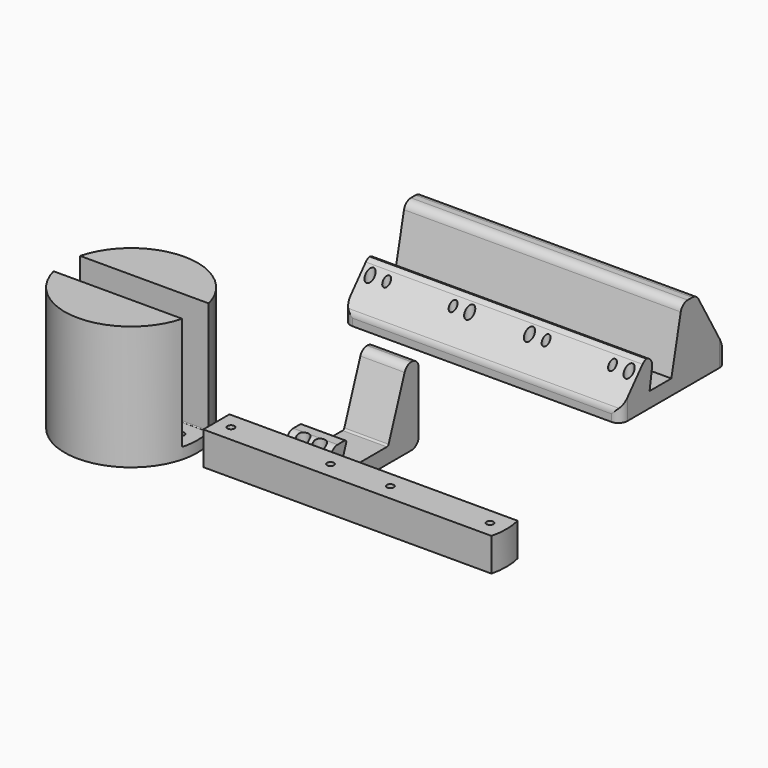
from build123d import *

# Parameters (mm, degrees)
F0_R            = 38.1
F1_DEPTH        = 71.12
F3_DEPTH        = 64.77
F4_R            = 2
F5_DEPTH        = 3.5
F5_FACE_R       = 2
F6_DEPTH        = 25.4
F7_R            = 2
F8_DEPTH        = 3.5
F9_DEPTH        = 6.351
F10_R           = 0.508
F11_R           = 2
F12_DEPTH       = 19.05
F13_W           = 158.75
F13_H           = 76.2
F13_R           = 2.5
F13_R_2         = 2
F14_DEPTH       = 6
F16_DEPTH       = 158.75
F17_T1_DEPTH    = 168.2889113945
F17_T3_DEPTH    = 170.280744219
F17_T5_DEPTH    = 31.4
F17_T7_DEPTH    = 165.5459461939
F17_T9_DEPTH    = 173.4270951792
F17_T11_DEPTH   = 179.186662319
F17_T13_DEPTH   = 188.398497554
F18_DEPTH       = 65.1210001
F20_DEPTH       = 25.4
F21_R           = 5.08
F22_R           = 1.27
F25_D           = 3.5
F25_DEPTH       = 25.4
F25_START       = 7.9337086
F25_CBORE_D     = 7
F25_CBORE_DEPTH = 7.112
F25_TIP         = 1.0515060833


# Not quite as in the source:
# - a fillet or chamfer that OpenCascade refuses, or shapes differently, is made with other operations: its cross-section is extruded or revolved along the edge and cut away or added


with BuildPart() as f1:
    # F0 (on Top) → F1 (new body)
    with BuildSketch(Plane.XY):
        with Locations((-43.8732802868, -98.4302014112)):
            Circle(F0_R)
    extrude(amount=F1_DEPTH)

    # F2 (on face) → F3 (cut)
    with BuildSketch(Plane.XY.offset(71.12)):
        with BuildLine():
            Line((-6.9831139142, -88.9052014112), (-80.7634466594, -88.9052014112))
            ThreePointArc((-80.7634466594, -88.9052014112), (-81.6696117146, -93.6294378677), (-81.9732802868, -98.4302014112))
            ThreePointArc((-81.9732802868, -98.4302014112), (-81.6696117146, -103.2309649548), (-80.7634466594, -107.9552014112))
            Line((-80.7634466594, -107.9552014112), (-6.9831139142, -107.9552014112))
            ThreePointArc((-6.9831139142, -107.9552014112), (-6.076948859, -103.2309649548), (-5.7732802868, -98.4302014112))
            ThreePointArc((-5.7732802868, -98.4302014112), (-6.076948859, -93.6294378677), (-6.9831139142, -88.9052014112))
        make_face()
    extrude(amount=-F3_DEPTH, mode=Mode.SUBTRACT)

    # F4 (on face) → F5 (cut)
    with BuildSketch(Plane(origin=(0, 0, 0), x_dir=(1, 0, 0), z_dir=(0, 0, -1))):
        Polygon((-75.9123819019, 98.4302014112), (-74.1803310944, 95.4302014112), (-70.7162294792, 95.4302014112), (-68.9841786717, 98.4302014112), (-70.7162294792, 101.4302014112), (-74.1803310944, 101.4302014112), align=None)
        with Locations((-72.4482802868, 98.4302014112)):
            Circle(F4_R, mode=Mode.SUBTRACT)
        Polygon((-17.0303310944, 95.4302014112), (-13.5662294792, 95.4302014112), (-11.8341786717, 98.4302014112), (-13.5662294792, 101.4302014112), (-17.0303310944, 101.4302014112), (-18.7623819019, 98.4302014112), align=None)
        with Locations((-15.2982802868, 98.4302014112)):
            Circle(F4_R, mode=Mode.SUBTRACT)
    extrude(amount=-F5_DEPTH, mode=Mode.SUBTRACT)

    # F5_face (on face) + F4 (on face) → F6 (cut)
    with BuildSketch(Plane(origin=(-72.4482802868, -98.4302014112, 0), x_dir=(1, 0, 0), z_dir=(0, 0, -1))):
        Circle(F5_FACE_R)
    with BuildSketch(Plane(origin=(0, 0, 0), x_dir=(1, 0, 0), z_dir=(0, 0, -1))):
        with Locations((-15.2982802868, 98.4302014112)):
            Circle(F4_R)
    extrude(amount=-F6_DEPTH, mode=Mode.SUBTRACT)

    # F7 (on face) → F8 (cut)
    with BuildSketch(Plane.XY.offset(6.35)):
        Polygon((-59.4591786717, -98.4302014112), (-61.1912294792, -95.4302014112), (-64.6553310944, -95.4302014112), (-66.3873819019, -98.4302014112), (-64.6553310944, -101.4302014112), (-61.1912294792, -101.4302014112), align=None)
        with Locations((-62.9232802868, -98.4302014112)):
            Circle(F7_R, mode=Mode.SUBTRACT)
        Polygon((-23.0912294792, -95.4302014112), (-26.5553310944, -95.4302014112), (-28.2873819019, -98.4302014112), (-26.5553310944, -101.4302014112), (-23.0912294792, -101.4302014112), (-21.3591786717, -98.4302014112), align=None)
        with Locations((-24.8232802868, -98.4302014112)):
            Circle(F7_R, mode=Mode.SUBTRACT)
    extrude(amount=-F8_DEPTH, mode=Mode.SUBTRACT)

    # F9 (cut, through all): faces of the model
    f9_faces = [f1.faces().sort_by_distance(p)[0] for p in [
        (-62.9232802868, -98.4302014112, 6.35),
        (-24.8232802868, -98.4302014112, 6.35),
    ]]
    extrude(f9_faces, amount=-F9_DEPTH, mode=Mode.SUBTRACT)

    # F10
    f10_edges = [f1.edges().sort_by_distance(p)[0] for p in [
        (-43.87328, -107.955201, 6.35),
        (-43.87328, -88.905201, 6.35),
    ]]
    fillet(f10_edges, radius=F10_R)


with BuildPart() as f12:
    # F11 (on Top) → F12 (new body)
    with BuildSketch(Plane.XY):
        with BuildLine():
            Line((170.2848374923, -89.0063627977), (4.9993881809, -89.0063627977))
            Line((4.9993881809, -89.0063627977), (4.9993881809, -107.8023627977))
            Line((4.9993881809, -107.8023627977), (170.2848374923, -107.8023627977))
            ThreePointArc((170.2848374923, -107.8023627977), (171.4621128366, -98.4043627977), (170.2848374923, -89.0063627977))
        make_face()
        with Locations((13.3471128366, -98.4043627977)):
            Circle(F11_R, mode=Mode.SUBTRACT)
        with Locations((70.4971128366, -98.4043627977)):
            Circle(F11_R, mode=Mode.SUBTRACT)
        with Locations((104.7871128366, -98.4043627977)):
            Circle(F11_R, mode=Mode.SUBTRACT)
        with Locations((161.9371128366, -98.4043627977)):
            Circle(F11_R, mode=Mode.SUBTRACT)
    extrude(amount=F12_DEPTH)


with BuildPart() as f14:
    # F13 (on Top) → F14 (new body)
    with BuildSketch(Plane.XY):
        with Locations((46.0346470964, 78.7849075437)):
            Rectangle(F13_W, F13_H)
        with Locations((-28.2603529036, 53.3849075437)):
            Circle(F13_R, mode=Mode.SUBTRACT)
        with Locations((-18.7353529036, 53.3849075437)):
            Circle(F13_R_2, mode=Mode.SUBTRACT)
        with Locations((19.3646470964, 53.3849075437)):
            Circle(F13_R_2, mode=Mode.SUBTRACT)
        with Locations((28.8896470964, 53.3849075437)):
            Circle(F13_R, mode=Mode.SUBTRACT)
        with Locations((63.1796470964, 53.3849075437)):
            Circle(F13_R, mode=Mode.SUBTRACT)
        with Locations((72.7046470964, 53.3849075437)):
            Circle(F13_R_2, mode=Mode.SUBTRACT)
        with Locations((110.8046470964, 53.3849075437)):
            Circle(F13_R_2, mode=Mode.SUBTRACT)
        with Locations((120.3296470964, 53.3849075437)):
            Circle(F13_R, mode=Mode.SUBTRACT)
    extrude(amount=F14_DEPTH)

    # F15 (on face) → F16 (join, through all)
    with BuildSketch(Plane.YZ.offset(125.4096470964)):
        Polygon((58.1746958196, 26.0015837848), (40.6849075437, 6), (116.8849075437, 6), (95.2580943704, 43.5221455991), (84.9392339587, 43.5221455991), (77.3075819016, 8.6959982291), (61.7218054831, 8.6959982291), (64.4090101123, 26.0015837848), align=None)
    extrude(amount=-F16_DEPTH)

    # F17: fillet of radius 5.08 on 10 edges, made by hand

    # F17_s2 → F17_t1 (cut)
    with BuildSketch(Plane.YZ.offset(-38.1098086008)):
        with BuildLine():
            ThreePointArc((40.6849075437, 4.0922177211), (41.0092121962, 5.878208136), (41.940719261, 7.436165086))
            Line((41.940719261, 7.436165086), (40.6849075437, 6))
            Line((40.6849075437, 6), (40.6849075437, 4.0922177211))
        make_face()
    extrude(amount=F17_T1_DEPTH, mode=Mode.SUBTRACT)

    # F17_s4 → F17_t3 (cut)
    with BuildSketch(Plane.YZ.offset(-39.1057250131)):
        with BuildLine():
            ThreePointArc((56.6566563808, 24.2655311497), (58.3809461675, 25.5472541478), (60.4808446634, 26.0015837848))
            Line((60.4808446634, 26.0015837848), (58.1746958196, 26.0015837848))
            Line((58.1746958196, 26.0015837848), (56.6566563808, 24.2655311497))
        make_face()
    extrude(amount=F17_T3_DEPTH, mode=Mode.SUBTRACT)

    # F17_s6 → F17_t5 (cut)
    with BuildSketch(Plane.XY.offset(-12.7)):
        with BuildLine():
            ThreePointArc((-33.3403529036, 45.7649075437), (-31.852455352, 42.1728050952), (-28.2603529036, 40.6849075437))
            Line((-28.2603529036, 40.6849075437), (-33.3403529036, 40.6849075437))
            Line((-33.3403529036, 40.6849075437), (-33.3403529036, 45.7649075437))
        make_face()
        with BuildLine():
            ThreePointArc((125.4096470964, 45.7649075437), (123.9217495448, 42.1728050952), (120.3296470964, 40.6849075437))
            Line((120.3296470964, 40.6849075437), (125.4096470964, 40.6849075437))
            Line((125.4096470964, 40.6849075437), (125.4096470964, 45.7649075437))
        make_face()
        with BuildLine():
            ThreePointArc((120.3296470964, 116.8849075437), (123.9217495448, 115.3970099921), (125.4096470964, 111.8049075437))
            Line((125.4096470964, 111.8049075437), (125.4096470964, 116.8849075437))
            Line((125.4096470964, 116.8849075437), (120.3296470964, 116.8849075437))
        make_face()
        with BuildLine():
            ThreePointArc((-28.2603529036, 116.8849075437), (-31.852455352, 115.3970099921), (-33.3403529036, 111.8049075437))
            Line((-33.3403529036, 111.8049075437), (-33.3403529036, 116.8849075437))
            Line((-33.3403529036, 116.8849075437), (-28.2603529036, 116.8849075437))
        make_face()
    extrude(amount=F17_T5_DEPTH, mode=Mode.SUBTRACT)

    # F17_s8 → F17_t7 (cut)
    with BuildSketch(Plane.YZ.offset(-36.7383260006)):
        with BuildLine():
            ThreePointArc((116.8849075437, 4.6408107612), (116.7122916498, 5.9538154202), (116.2061747742, 7.1775895781))
            Line((116.2061747742, 7.1775895781), (116.8849075437, 6))
            Line((116.8849075437, 6), (116.8849075437, 4.6408107612))
        make_face()
    extrude(amount=F17_T7_DEPTH, mode=Mode.SUBTRACT)

    # F17_s10 → F17_t9 (cut)
    with BuildSketch(Plane.YZ.offset(-40.6789004932)):
        with BuildLine():
            ThreePointArc((96.723942565, 40.978924416), (94.8642854158, 42.8406246766), (92.3226753345, 43.5221455991))
            Line((92.3226753345, 43.5221455991), (95.2580943704, 43.5221455991))
            Line((95.2580943704, 43.5221455991), (96.723942565, 40.978924416))
        make_face()
    extrude(amount=F17_T9_DEPTH, mode=Mode.SUBTRACT)

    # F17_s12 → F17_t11 (cut)
    with BuildSketch(Plane.YZ.offset(-43.5586840631)):
        with BuildLine():
            ThreePointArc((89.0265664225, 43.5221455991), (85.842043341, 42.4000759602), (84.0643142217, 39.5295521909))
            Line((84.0643142217, 39.5295521909), (84.9392339587, 43.5221455991))
            Line((84.9392339587, 43.5221455991), (89.0265664225, 43.5221455991))
        make_face()
    extrude(amount=F17_T11_DEPTH, mode=Mode.SUBTRACT)

    # F17_s14 → F17_t13 (cut)
    with BuildSketch(Plane.YZ.offset(-48.1646016806)):
        with BuildLine():
            ThreePointArc((63.4991524645, 20.1421046826), (62.3371697124, 24.2266288799), (58.4793106015, 26.0015837848))
            Line((58.4793106015, 26.0015837848), (64.4090101123, 26.0015837848))
            Line((64.4090101123, 26.0015837848), (63.4991524645, 20.1421046826))
        make_face()
    extrude(amount=F17_T13_DEPTH, mode=Mode.SUBTRACT)

    # F18 (cut, through all): faces of the model
    f18_faces = [f14.faces().sort_by_distance(p)[0] for p in [
        (-28.2603529036, 53.3849075437, 6),
        (-18.7353529036, 53.3849075437, 6),
        (63.1796470964, 53.3849075437, 6),
        (28.8896470964, 53.3849075437, 6),
        (120.3296470964, 53.3849075437, 6),
        (110.8046470964, 53.3849075437, 6),
        (19.3646470964, 53.3849075437, 6),
        (72.7046470964, 53.3849075437, 6),
    ]]
    extrude(f18_faces, amount=-F18_DEPTH, mode=Mode.SUBTRACT)


with BuildPart() as f20:
    # F19 (on Right) → F20 (new body)
    with BuildSketch(Plane.YZ):
        Polygon((-40.3678063909, -10.7832700619), (-46.846513316, -26.297595231), (-46.846513316, -35.187595231), (21.2055585506, -35.187595231), (21.2055585506, -26.297595231), (21.2055585506, 9.5046936209), (12.3155585506, 9.5046936209), (-0.7154089101, -26.297595231), (-35.8545589572, -26.297595231), (-30.2078063909, -10.7832700619), align=None)
    extrude(amount=F20_DEPTH)

    # F21
    f21_edges = [f20.edges().sort_by_distance(p)[0] for p in [
        (12.7, 12.315559, 9.504694),
        (12.7, 21.205559, 9.504694),
        (12.7, 21.205559, -35.187595),
        (12.7, -46.846513, -26.297595),
        (12.7, -40.367806, -10.78327),
    ]]
    fillet(f21_edges, radius=F21_R)

    # F22
    f22_edges = [f20.edges().sort_by_distance(p)[0] for p in [
        (12.7, -30.207806, -10.78327),
        (12.7, -35.854559, -26.297595),
        (12.7, -0.715409, -26.297595),
        (12.7, -46.846513, -35.187595),
    ]]
    fillet(f22_edges, radius=F22_R)

    # F25
    # its depths count from where the whole tool has entered the part; down to there all is cleared
    with Locations(Plane.XY.offset(-10.7832700619).offset(-F25_START)):
        with Locations((7.9375, -40.180884566), (17.4625, -40.180884566)):
            CounterBoreHole(F25_D / 2, F25_CBORE_D / 2, F25_CBORE_DEPTH, depth=F25_DEPTH)
            with Locations((0, 0, -(F25_DEPTH + F25_TIP / 2))):  # 118° drill point
                Cone(0, F25_D / 2, F25_TIP, mode=Mode.SUBTRACT)


solid = Compound([f1.part, f12.part, f14.part, f20.part])
